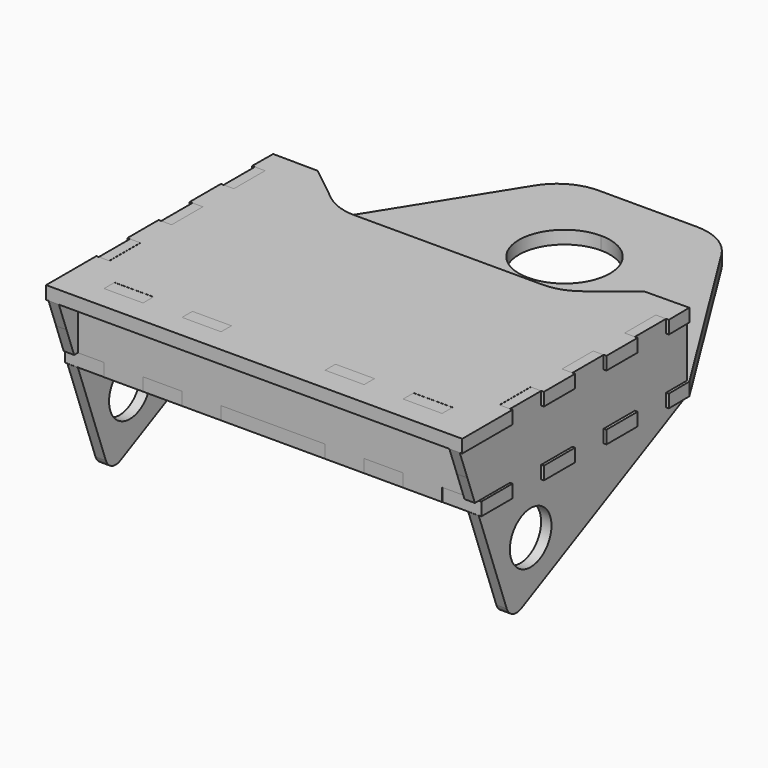
from build123d import *

# Parameters (mm, degrees)
F1_DEPTH = 5
F2_R     = 10
F2_W     = 14.9999479834
F2_H     = 5
F3_DEPTH = 4
F5_W     = 15
F5_H     = 5
F6_DEPTH = 5
F7_W     = 15
F7_H     = 5
F8_DEPTH = 5


# Not quite as in the source:
# - ends of sketch curves that miss each other by under 0.0002 mm in the source are joined


with BuildPart() as f1:
    # F0 (on Top) → F1 (new body)
    with BuildSketch(Plane.XY):
        with BuildLine():
            Line((-35.87501325, 70.5999788001), (-80, 0))
            Line((-80, 0), (-80.1117316498, -10.0001040331))
            Line((-80.1117316498, -10.0001040331), (-75.1117316498, -10.0001040331))
            Line((-75.1117316498, -10.0001040331), (-75.1117316498, -25.0001040331))
            Line((-75.1117316498, -25.0001040331), (-80.1117316498, -25.0001040331))
            Line((-80.1117316498, -25.0001040331), (-80.1117316498, -40.0001040331))
            Line((-80.1117316498, -40.0001040331), (-75.0558658249, -40.0000520166))
            Line((-75.0558658249, -40.0000520166), (-75.0558658249, -55.0000520166))
            Line((-75.0558658249, -55.0000520166), (-80.0558658249, -55.0000520166))
            Line((-80.0558658249, -55.0000520166), (-80.0558658249, -70.0000520166))
            Line((-80.0558658249, -70.0000520166), (-75, -70))
            Line((-75, -70), (-75, -85))
            Line((-75, -85), (-80, -85))
            Line((-80, -85), (-80, -100))
            Line((-80, -100), (-65, -100))
            Line((-65, -100), (-65, -95))
            Line((-65, -95), (-50, -95))
            Line((-50, -95), (-50, -100.0558658249))
            Line((-50, -100.0558658249), (-35.0000520166, -100.0558658249))
            Line((-35.0000520166, -100.0558658249), (-35.0000520166, -95.0558658249))
            Line((-35.0000520166, -95.0558658249), (-20.0000520166, -95.0558658249))
            Line((-20.0000520166, -95.0558658249), (-20.0000520166, -100.0558658249))
            Line((-20.0000520166, -100.0558658249), (0, -100.0558658249))
            Line((0, -100.0558658249), (20.0000520166, -100.0558658249))
            Line((20.0000520166, -100.0558658249), (20.0000520166, -95.0558658249))
            Line((20.0000520166, -95.0558658249), (35.0000520166, -95.0558658249))
            Line((35.0000520166, -95.0558658249), (35.0000520166, -100.0558658249))
            Line((35.0000520166, -100.0558658249), (50.0000520166, -100.0558658249))
            Line((50.0000520166, -100.0558658249), (50, -95))
            Line((50, -95), (65, -95))
            Line((65, -95), (65, -100))
            Line((65, -100), (80, -100))
            Line((80, -100), (80, -85))
            Line((80, -85), (75, -85))
            Line((75, -85), (75, -70))
            Line((75, -70), (80.0558658249, -70.0000520166))
            Line((80.0558658249, -70.0000520166), (80.0558658249, -55.0000520166))
            Line((80.0558658249, -55.0000520166), (75.0558658249, -55.0000520166))
            Line((75.0558658249, -55.0000520166), (75.0558658249, -40.0000520166))
            Line((75.0558658249, -40.0000520166), (80.1117316498, -40.0000520166))
            Line((80.1117316498, -40.0000520166), (80.1117316498, -25.0001040331))
            Line((80.1117316498, -25.0001040331), (75.1117316498, -25.0001040331))
            Line((75.1117316498, -25.0001040331), (75.1117316498, -10.0001040331))
            Line((75.1117316498, -10.0001040331), (80.1117316498, -10.0001040331))
            Line((80.1117316498, -10.0001040331), (80, 0))
            Line((80, 0), (35.87501325, 70.5999788001))
            ThreePointArc((35.87501325, 70.5999788001), (28.6104178177, 77.4928496249), (18.9150471699, 80))
            Line((18.9150471699, 80), (0, 80))
            Line((0, 80), (-18.9150471699, 80))
            ThreePointArc((-18.9150471699, 80), (-28.6104178177, 77.4928496249), (-35.87501325, 70.5999788001))
        make_face()
        with BuildLine():
            ThreePointArc((0, 22.5), (-17.5, 40), (0, 57.5))
            ThreePointArc((0, 57.5), (12.3743686708, 52.3743686708), (17.5, 40))
            ThreePointArc((17.5, 40), (12.3743686708, 27.6256313292), (0, 22.5))
        make_face(mode=Mode.SUBTRACT)
    extrude(amount=F1_DEPTH)


with BuildPart() as f3:
    # F2 (on face) → F3 (new body)
    with BuildSketch(Plane.YZ.offset(75.0558658249)):
        with BuildLine():
            Line((0, 0), (-10.0001040331, 0))
            Line((-10.0001040331, 0), (-10.0001040331, 5))
            Line((-10.0001040331, 5), (0, 5))
            Line((0, 5), (0, 25))
            Line((0, 25), (-10.0001040331, 25))
            Line((-10.0001040331, 25), (-10.0001040331, 30))
            Line((-10.0001040331, 30), (-25.0001040331, 30))
            Line((-25.0001040331, 30), (-25.0001040331, 25))
            Line((-25.0001040331, 25), (-40.0000520166, 25))
            Line((-40.0000520166, 25), (-40.0000520166, 30))
            Line((-40.0000520166, 30), (-55.0000520166, 30))
            Line((-55.0000520166, 30), (-55.0000520166, 25))
            Line((-55.0000520166, 25), (-70.0000520166, 25))
            Line((-70.0000520166, 25), (-70, 30))
            Line((-70, 30), (-85, 30))
            Line((-85, 30), (-85, 25))
            Line((-85, 25), (-100, 25))
            Line((-100, 25), (-109.1551216816, 25))
            Line((-109.1551216816, 25), (-105.5154193389, 15))
            Line((-105.5154193389, 15), (-101.8757169963, 5))
            Line((-101.8757169963, 5), (-85, 5))
            Line((-85, 5), (-85, 0))
            Line((-85, 0), (-100.0558658249, 0))
            Line((-100.0558658249, 0), (-86.5823112494, -37.0182869561))
            ThreePointArc((-86.5823112494, -37.0182869561), (-83.7350152341, -39.9528800303), (-79.6497378177, -39.7813004839))
            Line((-79.6497378177, -39.7813004839), (0, 0))
        make_face()
        with Locations((-75.0734061003, -17.5903327763)):
            Circle(F2_R, mode=Mode.SUBTRACT)
        Polygon((-70.0000520166, 5), (-55.0000520166, 5), (-55.0000520166, 0), (-70, 0), align=None, mode=Mode.SUBTRACT)
        with Locations((-32.5000780248, 2.5)):
            Rectangle(F2_W, F2_H, mode=Mode.SUBTRACT)
    extrude(amount=F3_DEPTH)


with BuildPart() as f4_1:
    # F4: instance of F3
    add(f3.part.mirror(Plane.YZ))


with BuildPart() as f6:
    # F5 (on face) → F6 (new body)
    with BuildSketch(Plane.XY.offset(25)):
        with BuildLine():
            Line((-62.7239066089, -0.1930266336), (-80, 0))
            Line((-80, 0), (-80.1117316498, -10.0001040331))
            Line((-80.1117316498, -10.0001040331), (-75.1117316498, -10.0001040331))
            Line((-75.1117316498, -10.0001040331), (-75.1117316498, -25.0001040331))
            Line((-75.1117316498, -25.0001040331), (-80.1117316498, -25.0001040331))
            Line((-80.1117316498, -25.0001040331), (-80.1117316498, -40.0001040331))
            Line((-80.1117316498, -40.0001040331), (-75.0558658249, -40.0000520166))
            Line((-75.0558658249, -40.0000520166), (-75.0558658249, -55.0000520166))
            Line((-75.0558658249, -55.0000520166), (-80.0558658249, -55.0000520166))
            Line((-80.0558658249, -55.0000520166), (-80.0558658249, -70.0000520166))
            Line((-80.0558658249, -70.0000520166), (-75, -70))
            Line((-75, -70), (-75, -85))
            Line((-75, -85), (-80, -85))
            Line((-80, -85), (-80, -100))
            Line((-80, -100), (-80, -109.1551216816))
            Line((-80, -109.1551216816), (-79.0558658249, -109.1551216816))
            Line((-79.0558658249, -109.1551216816), (-75.0558658249, -109.1551216816))
            Line((-75.0558658249, -109.1551216816), (80, -109.1551216816))
            Line((80, -109.1551216816), (80, -100))
            Line((80, -100), (80, -85))
            Line((80, -85), (75, -85))
            Line((75, -85), (75, -70))
            Line((75, -70), (80.0558658249, -70.0000520166))
            Line((80.0558658249, -70.0000520166), (80.0558658249, -55.0000520166))
            Line((80.0558658249, -55.0000520166), (75.0558658249, -55.0000520166))
            Line((75.0558658249, -55.0000520166), (75.0558658249, -40.0000520166))
            Line((75.0558658249, -40.0000520166), (80.1117316498, -40.0000520166))
            Line((80.1117316498, -40.0000520166), (80.1117316498, -25.0001040331))
            Line((80.1117316498, -25.0001040331), (75.1117316498, -25.0001040331))
            Line((75.1117316498, -25.0001040331), (75.1117316498, -10.0001040331))
            Line((75.1117316498, -10.0001040331), (80.1117316498, -10.0001040331))
            Line((80.1117316498, -10.0001040331), (80, 0))
            Line((80, 0), (62.7239066089, -0.1930266336))
            Line((62.7239066089, -0.1930266336), (48.5575296192, -11.4846958312))
            ThreePointArc((48.5575296192, -11.4846958312), (42.6948235789, -14.7235020195), (36.0915396388, -15.8450317106))
            Line((36.0915396388, -15.8450317106), (0, -15.8450317106))
            Line((0, -15.8450317106), (-36.0915396388, -15.8450317106))
            ThreePointArc((-36.0915396388, -15.8450317106), (-42.6948235789, -14.7235020195), (-48.5575296192, -11.4846958312))
            Line((-48.5575296192, -11.4846958312), (-62.7239066089, -0.1930266336))
        make_face()
        Polygon((-50, -100.0558658249), (-65, -100), (-65, -95), (-50, -95), align=None, mode=Mode.SUBTRACT)
        with Locations((-27.5000520166, -97.5558658249)):
            Rectangle(F5_W, F5_H, mode=Mode.SUBTRACT)
        with Locations((27.5000520166, -97.5558658249)):
            Rectangle(F5_W, F5_H, mode=Mode.SUBTRACT)
        Polygon((65, -100), (50.0000520166, -100.0558658249), (50, -95), (65, -95), align=None, mode=Mode.SUBTRACT)
    extrude(amount=F6_DEPTH)


with BuildPart() as f8:
    # F7 (on face) → F8 (new body)
    with BuildSketch(Plane.XZ.offset(95.0558658249)):
        with BuildLine():
            Line((-75.0558658249, 5), (-65, 5))
            Line((-65, 5), (-65, 0))
            Line((-65, 0), (-50, 0))
            add(Edge.make_bspline(
                [(-50, 5), (-50, 3.3333333333), (-50, 1.6666666667), (-50, 0)],
                knots=[0, 0, 0, 0, 1, 1, 1, 1], degree=3))
            Line((-50, 5), (-35.0000520166, 5))
            Line((-35.0000520166, 5), (-35.0000520166, 0))
            Line((-35.0000520166, 0), (-20.0000520166, 0))
            Line((-20.0000520166, 0), (-20.0000520166, 5))
            Line((-20.0000520166, 5), (20.0000520166, 5))
            Line((20.0000520166, 5), (20.0000520166, 0))
            Line((20.0000520166, 0), (35.0000520166, 0))
            Line((35.0000520166, 0), (35.0000520166, 5))
            Line((35.0000520166, 5), (50, 5))
            add(Edge.make_bspline(
                [(50, 5), (50, 3.3333333333), (50, 1.6666666667), (50, 0)],
                knots=[0, 0, 0, 0, 1, 1, 1, 1], degree=3))
            Line((50, 0), (65, 0))
            Line((65, 0), (65, 5))
            Line((65, 5), (75.0558658249, 5))
            Line((75.0558658249, 5), (75.0558658249, 25))
            Line((75.0558658249, 25), (65, 25))
            Line((65, 25), (65, 30))
            Line((65, 30), (50, 30))
            add(Edge.make_bspline(
                [(50, 30), (50, 28.3333333333), (50, 26.6666666667), (50, 25)],
                knots=[0, 0, 0, 0, 1, 1, 1, 1], degree=3))
            Line((50, 25), (35.0000520166, 25))
            Line((35.0000520166, 25), (35.0000520166, 30))
            Line((35.0000520166, 30), (20.0000520166, 30))
            Line((20.0000520166, 30), (20.0000520166, 25))
            Line((20.0000520166, 25), (-20.0000520166, 25))
            Line((-20.0000520166, 25), (-35.0000520166, 25))
            Line((-35.0000520166, 25), (-50, 25))
            add(Edge.make_bspline(
                [(-50, 30), (-50, 28.3333333333), (-50, 26.6666666667), (-50, 25)],
                knots=[0, 0, 0, 0, 1, 1, 1, 1], degree=3))
            Line((-50, 30), (-65, 30))
            Line((-65, 30), (-65, 25))
            Line((-65, 25), (-75.0558658249, 25))
            Line((-75.0558658249, 25), (-75.0558658249, 5))
        make_face()
        with Locations((-27.5000520166, 27.5)):
            Rectangle(F7_W, F7_H)
    extrude(amount=F8_DEPTH)


solid = Compound([f1.part, f3.part, f4_1.part, f6.part, f8.part])
